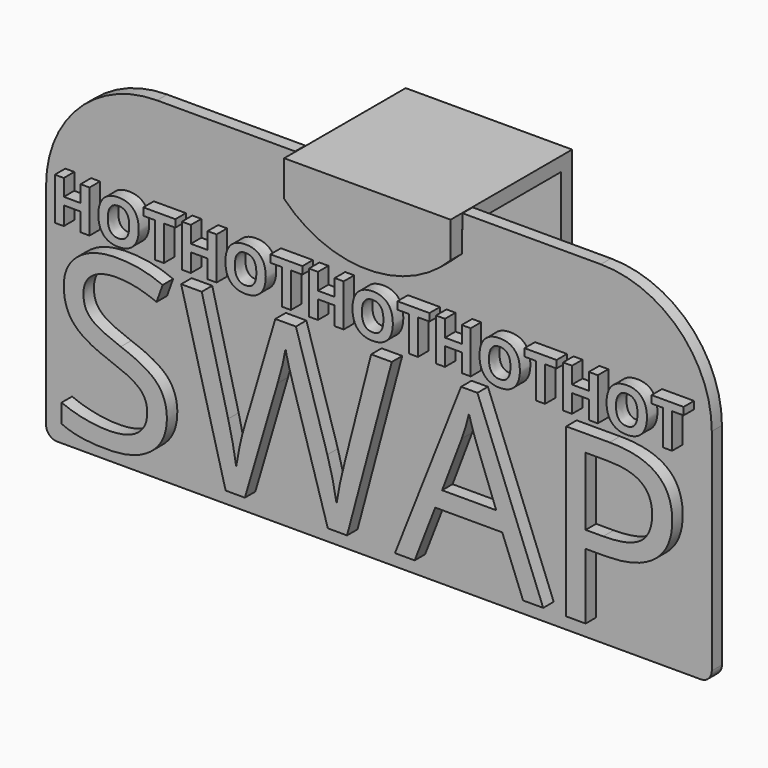
from build123d import *

# Parameters (mm, degrees)
F1_DEPTH       = 2.9
F2_TEXT_SIZE   = 13.5915779678
F2_TEXT_SIZE_2 = 53.6332338765
F3_DEPTH       = 3
F6_DEPTH       = 19.05
F7_W           = 38.3215658367
F7_H           = 3.3903783083
F8_DEPTH       = 25.4
F10_DEPTH      = 25.4


# Not quite as in the source:
# - Text() gives the source's letters only with a copy of the font that has no kerning and outlines rounded to 1/6400 em; it was checked with that copy


with BuildPart() as f1:
    # F0 (on Front) → F1 (new body)
    with BuildSketch(Plane.XZ):
        with BuildLine():
            Line((-149.86, 0), (-2.54, 0))
            ThreePointArc((-2.54, 0), (-0.7439487758, 0.7439487758), (0, 2.54))
            Line((0, 2.54), (0, 50.8))
            ThreePointArc((0, 50.8), (-7.4394877579, 68.7605122421), (-25.4, 76.2))
            Line((-25.4, 76.2), (-127, 76.2))
            ThreePointArc((-127, 76.2), (-144.9605122421, 68.7605122421), (-152.4, 50.8))
            Line((-152.4, 50.8), (-152.4, 2.54))
            ThreePointArc((-152.4, 2.54), (-151.6560512242, 0.7439487758), (-149.86, 0))
        make_face()
    extrude(amount=F1_DEPTH)

    # F2 (on face) → F3 (join)
    with BuildSketch(Plane.XZ.offset(2.9)):
        with Locations((-149.225, 45.915202165)):
            Text('HOTHOTHOTHOTHOT', F2_TEXT_SIZE, font='Open Sans', font_style=FontStyle.BOLD, text_align=(TextAlign.LEFT, TextAlign.BOTTOM))
        with Locations((-149.225, 4.6663857065)):
            Text('SWAP', F2_TEXT_SIZE_2, font='Open Sans', text_align=(TextAlign.LEFT, TextAlign.BOTTOM))
    extrude(amount=F3_DEPTH)

    # F7 (on face) → F8 (cut)
    with BuildSketch(Plane.XZ.offset(2.9)):
        with Locations((-76.2233454734, 74.5048108459)):
            Rectangle(F7_W, F7_H)
    extrude(amount=-F8_DEPTH, mode=Mode.SUBTRACT)


with BuildPart() as f6:
    # F5 (on offset) → F6 (new body, symmetric)
    with BuildSketch(Plane.YZ.offset(-76.2)):
        Polygon((28.575, 76.2068778276), (-6.2027284876, 76.2068778276), (-6.2027284876, 59.8316267133), (-2.9676526319, 59.8316267133), (-2.9, 72.9831904173), (25.4, 72.9831904173), (25.4, 55.2043892775), (28.575, 55.2043892775), align=None)
    extrude(amount=F6_DEPTH, both=True)

    # F9 (on face) → F10 (cut)
    with BuildSketch(Plane.XZ.offset(6.2027284876)):
        with BuildLine():
            ThreePointArc((-57.15, 68.0192522705), (-76.2, 59.9735156185), (-95.25, 68.0192522705))
            Line((-95.25, 68.0192522705), (-97.9798510671, 68.0192522705))
            Line((-97.9798510671, 68.0192522705), (-97.9798510671, 57.475887239))
            Line((-97.9798510671, 57.475887239), (-55.1781691611, 57.475887239))
            Line((-55.1781691611, 57.475887239), (-55.1781691611, 68.5631856322))
            Line((-55.1781691611, 68.5631856322), (-57.15, 68.0192522705))
        make_face()
    extrude(amount=-F10_DEPTH, mode=Mode.SUBTRACT)


solid = Compound([f1.part, f6.part])
